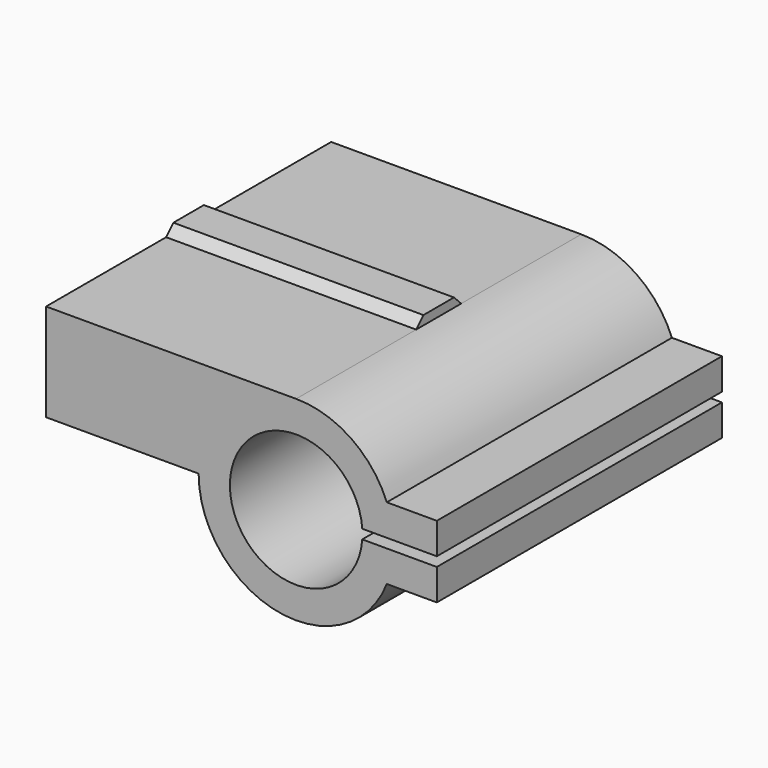
from build123d import *

# Parameters (mm, degrees)
F1_DEPTH = 57
F3_DEPTH = 40


# Not quite as in the source:
# - a feature of the source that left no trace in its solid (it failed there, or was rolled back) is left out


with BuildPart() as f1:
    # F0 (on Front) → F1 (new body)
    with BuildSketch(Plane.XZ):
        with BuildLine():
            ThreePointArc((-15.6, 0), (-11.0308657865, 11.0308657865), (0, 15.6))
            Line((0, 15.6), (-40, 15.6))
            Line((-40, 15.6), (-40, 0))
            Line((-40, 0), (-15.6, 0))
        make_face()
        with BuildLine():
            ThreePointArc((10.5734336902, -0.75), (-10.6, 0), (10.5734336902, 0.75))
            Line((10.5734336902, 0.75), (15.5819607239, 0.75))
            ThreePointArc((15.5819607239, 0.75), (15.2481384312, 3.2945825812), (14.5016378385, 5.75))
            ThreePointArc((14.5016378385, 5.75), (8.765272386, 12.9046503246), (0, 15.6))
            ThreePointArc((0, 15.6), (-11.0308657865, 11.0308657865), (-15.6, 0))
            ThreePointArc((-15.6, 0), (-2.9269822103, -15.3229492964), (14.5016378385, -5.75))
            ThreePointArc((14.5016378385, -5.75), (15.2481384312, -3.2945825812), (15.5819607239, -0.75))
            Line((15.5819607239, -0.75), (10.5734336902, -0.75))
        make_face()
        with BuildLine():
            ThreePointArc((14.5016378385, 5.75), (15.2481384312, 3.2945825812), (15.5819607239, 0.75))
            Line((15.5819607239, 0.75), (22.5016378385, 0.75))
            Line((22.5016378385, 0.75), (22.5016378385, 5.75))
            Line((22.5016378385, 5.75), (14.5016378385, 5.75))
        make_face()
        with BuildLine():
            Line((22.5016378385, -0.75), (15.5819607239, -0.75))
            ThreePointArc((15.5819607239, -0.75), (15.2481384312, -3.2945825812), (14.5016378385, -5.75))
            Line((14.5016378385, -5.75), (22.5016378385, -5.75))
            Line((22.5016378385, -5.75), (22.5016378385, -0.75))
        make_face()
    extrude(amount=F1_DEPTH)

    # F2 (on face) → F3 (join)
    with BuildSketch(Plane(origin=(-40, 0, 0), x_dir=(0, -1, 0), z_dir=(-1, 0, 0))):
        Polygon((25.45, 17.055), (24, 15.6), (33, 15.6), (31.55, 17.055), align=None)
    extrude(amount=-F3_DEPTH)


solid = f1.part
